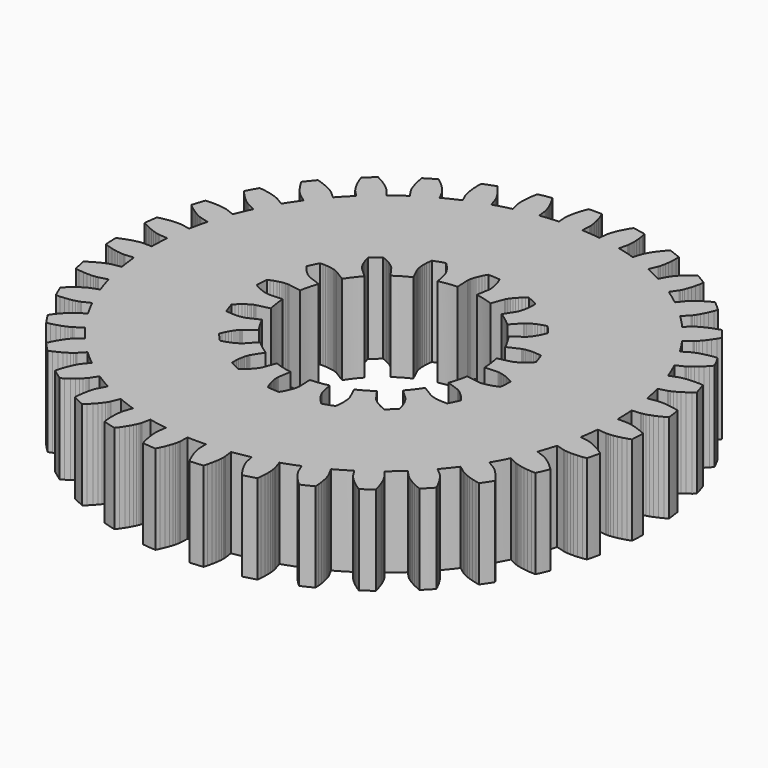
from build123d import *

# Parameters (mm, degrees)
F1_DEPTH = 5


# Not quite as in the source:
# - ends of sketch curves that miss each other by under 0.0002 mm in the source are joined


with BuildPart() as f1:
    # F0 (on Top) → F1 (new body)
    with BuildSketch(Plane.XY):
        with BuildLine():
            Line((10.175022, 8.940518), (9.814956, 8.623606))
            ThreePointArc((9.814956, 8.623606), (9.4680953178, 9.0024281141), (9.1066227348, 9.3673337267))
            Line((9.1066227348, 9.3673337267), (9.440701, 9.711531))
            Line((9.440701, 9.711531), (9.452089, 9.724074))
            Line((9.452089, 9.724074), (9.484545, 9.763184))
            Line((9.484545, 9.763184), (9.535389, 9.830931))
            Line((9.535389, 9.830931), (9.601788, 9.929185))
            Line((9.601788, 9.929185), (9.680771, 10.059599))
            Line((9.680771, 10.059599), (9.769248, 10.223605))
            Line((9.769248, 10.223605), (9.864016, 10.422403))
            Line((9.864016, 10.422403), (9.961783, 10.656955))
            Line((9.961783, 10.656955), (10.035983, 10.863432))
            ThreePointArc((10.035983, 10.863432), (9.7595522621, 11.1120973665), (9.4769619966, 11.3537399959))
            Line((9.4769619966, 11.3537399959), (9.281924, 11.253248))
            Line((9.281924, 11.253248), (9.062124, 11.125729))
            Line((9.062124, 11.125729), (8.877382, 11.005845))
            Line((8.877382, 11.005845), (8.726315, 10.896737))
            Line((8.726315, 10.896737), (8.607314, 10.801421))
            Line((8.607314, 10.801421), (8.518558, 10.722776))
            Line((8.518558, 10.722776), (8.45802, 10.663532))
            Line((8.45802, 10.663532), (8.423477, 10.626253))
            Line((8.423477, 10.626253), (8.412526, 10.613326))
            Line((8.412526, 10.613326), (8.114834, 10.237215))
            ThreePointArc((8.114834, 10.237215), (7.7059057986, 10.5480145502), (7.285085742, 10.8425126154))
            Line((7.285085742, 10.8425126154), (7.552337, 11.240831))
            Line((7.552337, 11.240831), (7.561302, 11.255206))
            Line((7.561302, 11.255206), (7.586253, 11.299482))
            Line((7.586253, 11.299482), (7.624183, 11.375219))
            Line((7.624183, 11.375219), (7.671971, 11.48375))
            Line((7.671971, 11.48375), (7.726399, 11.626171))
            Line((7.726399, 11.626171), (7.784169, 11.80334))
            Line((7.784169, 11.80334), (7.841917, 12.015864))
            Line((7.841917, 12.015864), (7.896232, 12.264104))
            Line((7.896232, 12.264104), (7.932372, 12.480512))
            ThreePointArc((7.932372, 12.480512), (7.6159827615, 12.6758223102), (7.2947870577, 12.8631231018))
            Line((7.2947870577, 12.8631231018), (7.120826, 12.72942))
            Line((7.120826, 12.72942), (6.927328, 12.564704))
            Line((6.927328, 12.564704), (6.766962, 12.41376))
            Line((6.766962, 12.41376), (6.637804, 12.279431))
            Line((6.637804, 12.279431), (6.537735, 12.164398))
            Line((6.537735, 12.164398), (6.464448, 12.07117))
            Line((6.464448, 12.07117), (6.415461, 12.002068))
            Line((6.415461, 12.002068), (6.38813, 11.95922))
            Line((6.38813, 11.95922), (6.379663, 11.944546))
            Line((6.379663, 11.944546), (6.153912, 11.521324))
            ThreePointArc((6.153912, 11.521324), (5.6960599686, 11.7541118719), (5.2294179645, 11.9687369187))
            Line((5.2294179645, 11.9687369187), (5.421252, 12.408373))
            Line((5.421252, 12.408373), (5.427506, 12.424118))
            Line((5.427506, 12.424118), (5.444151, 12.472138))
            Line((5.444151, 12.472138), (5.467948, 12.553431))
            Line((5.467948, 12.553431), (5.495588, 12.66875))
            Line((5.495588, 12.66875), (5.523711, 12.818601))
            Line((5.523711, 12.818601), (5.548918, 13.003238))
            Line((5.548918, 13.003238), (5.567791, 13.222658))
            Line((5.567791, 13.222658), (5.576908, 13.476607))
            Line((5.576908, 13.476607), (5.573826, 13.69599))
            ThreePointArc((5.573826, 13.69599), (5.2276470646, 13.8316685737), (4.8781689182, 13.9586077655))
            Line((4.8781689182, 13.9586077655), (4.730878, 13.795992))
            Line((4.730878, 13.795992), (4.569901, 13.599372))
            Line((4.569901, 13.599372), (4.439063, 13.422219))
            Line((4.439063, 13.422219), (4.335967, 13.266987))
            Line((4.335967, 13.266987), (4.258046, 13.135935))
            Line((4.258046, 13.135935), (4.202583, 13.031118))
            Line((4.202583, 13.031118), (4.166722, 12.95438))
            Line((4.166722, 12.95438), (4.147481, 12.90734))
            Line((4.147481, 12.90734), (4.14177, 12.891391))
            Line((4.14177, 12.891391), (3.995216, 12.43466))
            ThreePointArc((3.995216, 12.43466), (3.5031563536, 12.5819548058), (3.0056908928, 12.7098085461))
            Line((3.0056908928, 12.7098085461), (3.115942, 13.176633))
            Line((3.115942, 13.176633), (3.119284, 13.193242))
            Line((3.119284, 13.193242), (3.127087, 13.243462))
            Line((3.127087, 13.243462), (3.135986, 13.327697))
            Line((3.135986, 13.327697), (3.142591, 13.446099))
            Line((3.142591, 13.446099), (3.143506, 13.598563))
            Line((3.143506, 13.598563), (3.135339, 13.784734))
            Line((3.135339, 13.784734), (3.11473, 14.003998))
            Line((3.11473, 14.003998), (3.078356, 14.255493))
            Line((3.078356, 14.255493), (3.036151, 14.470801))
            ThreePointArc((3.036151, 14.470801), (2.6713088383, 14.5424859858), (2.3047810753, 14.6049834777))
            Line((2.3047810753, 14.6049834777), (2.188894, 14.418681))
            Line((2.188894, 14.418681), (2.065611, 14.196477))
            Line((2.065611, 14.196477), (1.968508, 13.998809))
            Line((1.968508, 13.998809), (1.894786, 13.827663))
            Line((1.894786, 13.827663), (1.841518, 13.684804))
            Line((1.841518, 13.684804), (1.805662, 13.571769))
            Line((1.805662, 13.571769), (1.784079, 13.48986))
            Line((1.784079, 13.48986), (1.773547, 13.440141))
            Line((1.773547, 13.440141), (1.770775, 13.423428))
            Line((1.770775, 13.423428), (1.708129, 12.947869))
            ThreePointArc((1.708129, 12.947869), (1.197676295, 13.0049359248), (0.6853760059, 13.0419091124))
            Line((0.6853760059, 13.0419091124), (0.710501, 13.520918))
            Line((0.710501, 13.520918), (0.710824, 13.537856))
            Line((0.710824, 13.537856), (0.709534, 13.588662))
            Line((0.709534, 13.588662), (0.703249, 13.673133))
            Line((0.703249, 13.673133), (0.688607, 13.790811))
            Line((0.688607, 13.790811), (0.662283, 13.940989))
            Line((0.662283, 13.940989), (0.621006, 14.122709))
            Line((0.621006, 14.122709), (0.561577, 14.33477))
            Line((0.561577, 14.33477), (0.480881, 14.575729))
            Line((0.480881, 14.575729), (0.400909, 14.78004))
            ThreePointArc((0.400909, 14.78004), (0.0291305244, 14.7854284308), (-0.3426659885, 14.7814755044))
            Line((-0.3426659885, 14.7814755044), (-0.423425, 14.577474))
            Line((-0.423425, 14.577474), (-0.505051, 14.336829))
            Line((-0.505051, 14.336829), (-0.565298, 14.124999))
            Line((-0.565298, 14.124999), (-0.607276, 13.94344))
            Line((-0.607276, 13.94344), (-0.63418, 13.793365))
            Line((-0.63418, 13.793365), (-0.649276, 13.675744))
            Line((-0.649276, 13.675744), (-0.655887, 13.591298))
            Line((-0.655887, 13.591298), (-0.657373, 13.540497))
            Line((-0.657373, 13.540497), (-0.657115, 13.523557))
            Line((-0.657115, 13.523557), (-0.63384, 13.044455))
            ThreePointArc((-0.63384, 13.044455), (-1.1462789677, 13.0094602448), (-1.6569479451, 12.9543645706))
            Line((-1.6569479451, 12.9543645706), (-1.717758, 13.430161))
            Line((-1.717758, 13.430161), (-1.720465, 13.446885))
            Line((-1.720465, 13.446885), (-1.730806, 13.496645))
            Line((-1.730806, 13.496645), (-1.752072, 13.578636))
            Line((-1.752072, 13.578636), (-1.787491, 13.691808))
            Line((-1.787491, 13.691808), (-1.840208, 13.834872))
            Line((-1.840208, 13.834872), (-1.913269, 14.006302))
            Line((-1.913269, 14.006302), (-2.009608, 14.204343))
            Line((-2.009608, 14.204343), (-2.132032, 14.427021))
            Line((-2.132032, 14.427021), (-2.247199, 14.61377))
            ThreePointArc((-2.247199, 14.61377), (-2.6139651037, 14.552687637), (-2.9790810776, 14.4824113773))
            Line((-2.9790810776, 14.4824113773), (-3.022117, 14.267268))
            Line((-3.022117, 14.267268), (-3.059462, 14.015915))
            Line((-3.059462, 14.015915), (-3.080918, 13.796732))
            Line((-3.080918, 13.796732), (-3.089802, 13.610595))
            Line((-3.089802, 13.610595), (-3.089477, 13.458128))
            Line((-3.089477, 13.458128), (-3.083328, 13.339702))
            Line((-3.083328, 13.339702), (-3.074755, 13.255432))
            Line((-3.074755, 13.255432), (-3.067145, 13.205183))
            Line((-3.067145, 13.205183), (-3.063867, 13.188561))
            Line((-3.063867, 13.188561), (-2.95542, 12.721315))
            ThreePointArc((-2.95542, 12.721315), (-3.4533751691, 12.595382232), (-3.9459998274, 12.4499884548))
            Line((-3.9459998274, 12.4499884548), (-4.090789, 12.907281))
            Line((-4.090789, 12.907281), (-4.096438, 12.923253))
            Line((-4.096438, 12.923253), (-4.115498, 12.970366))
            Line((-4.115498, 12.970366), (-4.151063, 13.047242))
            Line((-4.151063, 13.047242), (-4.20612, 13.152272))
            Line((-4.20612, 13.152272), (-4.283535, 13.283624))
            Line((-4.283535, 13.283624), (-4.386031, 13.439253))
            Line((-4.386031, 13.439253), (-4.516184, 13.61691))
            Line((-4.516184, 13.61691), (-4.676401, 13.81415))
            Line((-4.676401, 13.81415), (-4.823063, 13.977333))
            ThreePointArc((-4.823063, 13.977333), (-5.1730282225, 13.8517440222), (-5.5197280986, 13.7174032452))
            Line((-5.5197280986, 13.7174032452), (-5.523658, 13.498033))
            Line((-5.523658, 13.498033), (-5.515521, 13.244051))
            Line((-5.515521, 13.244051), (-5.497495, 13.024559))
            Line((-5.497495, 13.024559), (-5.473001, 12.839827))
            Line((-5.473001, 12.839827), (-5.445457, 12.689868))
            Line((-5.445457, 12.689868), (-5.418262, 12.574443))
            Line((-5.418262, 12.574443), (-5.394779, 12.493059))
            Line((-5.394779, 12.493059), (-5.378319, 12.444975))
            Line((-5.378319, 12.444975), (-5.372126, 12.429207))
            Line((-5.372126, 12.429207), (-5.181991, 11.988833))
            ThreePointArc((-5.181991, 11.988833), (-5.6494579891, 11.7760109862), (-6.1082050738, 11.5449921396))
            Line((-6.1082050738, 11.5449921396), (-6.33232, 11.969083))
            Line((-6.33232, 11.969083), (-6.340731, 11.983789))
            Line((-6.340731, 11.983789), (-6.367896, 12.026742))
            Line((-6.367896, 12.026742), (-6.416616, 12.096033))
            Line((-6.416616, 12.096033), (-6.489543, 12.189544))
            Line((-6.489543, 12.189544), (-6.589167, 12.304962))
            Line((-6.589167, 12.304962), (-6.717805, 12.439788))
            Line((-6.717805, 12.439788), (-6.877588, 12.59135))
            Line((-6.877588, 12.59135), (-7.070449, 12.756812))
            Line((-7.070449, 12.756812), (-7.243891, 12.891186))
            ThreePointArc((-7.243891, 12.891186), (-7.5658077628, 12.7051265282), (-7.8829488792, 12.5110388081))
            Line((-7.8829488792, 12.5110388081), (-7.847645, 12.294493))
            Line((-7.847645, 12.294493), (-7.794289, 12.046045))
            Line((-7.794289, 12.046045), (-7.737361, 11.833299))
            Line((-7.737361, 11.833299), (-7.680276, 11.655909))
            Line((-7.680276, 11.655909), (-7.626398, 11.513279))
            Line((-7.626398, 11.513279), (-7.579029, 11.404564))
            Line((-7.579029, 11.404564), (-7.541392, 11.328681))
            Line((-7.541392, 11.328681), (-7.516612, 11.284309))
            Line((-7.516612, 11.284309), (-7.507702, 11.2699))
            Line((-7.507702, 11.2699), (-7.241991, 10.870553))
            ThreePointArc((-7.241991, 10.870553), (-7.6639444746, 10.5776816964), (-8.0740691019, 10.2684631297))
            Line((-8.0740691019, 10.2684631297), (-8.370307, 10.645721))
            Line((-8.370307, 10.645721), (-8.381209, 10.658689))
            Line((-8.381209, 10.658689), (-8.415607, 10.696101))
            Line((-8.415607, 10.696101), (-8.475917, 10.755579))
            Line((-8.475917, 10.755579), (-8.564368, 10.834565))
            Line((-8.564368, 10.834565), (-8.683, 10.93034))
            Line((-8.683, 10.93034), (-8.833645, 11.040031))
            Line((-8.833645, 11.040031), (-9.017923, 11.160627))
            Line((-9.017923, 11.160627), (-9.237229, 11.288993))
            Line((-9.237229, 11.288993), (-9.431877, 11.390238))
            ThreePointArc((-9.431877, 11.390238), (-9.7153981255, 11.1496881714), (-9.9927868685, 10.9020918563))
            Line((-9.9927868685, 10.9020918563), (-9.919384, 10.69533))
            Line((-9.919384, 10.69533), (-9.822524, 10.460402))
            Line((-9.822524, 10.460402), (-9.728524, 10.26124))
            Line((-9.728524, 10.26124), (-9.640681, 10.096893))
            Line((-9.640681, 10.096893), (-9.562201, 9.966175))
            Line((-9.562201, 9.966175), (-9.496183, 9.867666))
            Line((-9.496183, 9.867666), (-9.445601, 9.799723))
            Line((-9.445601, 9.799723), (-9.413296, 9.760488))
            Line((-9.413296, 9.760488), (-9.401957, 9.747901))
            Line((-9.401957, 9.747901), (-9.069209, 9.402417))
            ThreePointArc((-9.069209, 9.402417), (-9.4320875894, 9.038909449), (-9.7804084177, 8.6614293705))
            Line((-9.7804084177, 8.6614293705), (-10.139248, 8.979729))
            Line((-10.139248, 8.979729), (-10.152289, 8.990542))
            Line((-10.152289, 8.990542), (-10.192815, 9.021211))
            Line((-10.192815, 9.021211), (-10.262776, 9.068964))
            Line((-10.262776, 9.068964), (-10.36391, 9.130888))
            Line((-10.36391, 9.130888), (-10.497736, 9.203941))
            Line((-10.497736, 9.203941), (-10.665546, 9.28497))
            Line((-10.665546, 9.28497), (-10.868396, 9.370724))
            Line((-10.868396, 9.370724), (-11.107098, 9.457869))
            Line((-11.107098, 9.457869), (-11.316696, 9.522731))
            ThreePointArc((-11.316696, 9.522731), (-11.5527092579, 9.2354223258), (-11.7814302901, 8.9422752205))
            Line((-11.7814302901, 8.9422752205), (-11.672288, 8.751942))
            Line((-11.672288, 8.751942), (-11.535036, 8.538085))
            Line((-11.535036, 8.538085), (-11.406985, 8.358908))
            Line((-11.406985, 8.358908), (-11.291209, 8.212888))
            Line((-11.291209, 8.212888), (-11.19065, 8.098283))
            Line((-11.19065, 8.098283), (-11.108103, 8.013145))
            Line((-11.108103, 8.013145), (-11.046202, 7.955325))
            Line((-11.046202, 7.955325), (-11.007411, 7.92249))
            Line((-11.007411, 7.92249), (-10.994006, 7.91213))
            Line((-10.994006, 7.91213), (-10.604918, 7.631612))
            ThreePointArc((-10.604918, 7.631612), (-10.8970576132, 7.2091516286), (-11.1723789546, 6.7755429724))
            Line((-11.1723789546, 6.7755429724), (-11.582286, 7.024654))
            Line((-11.582286, 7.024654), (-11.597049, 7.032965))
            Line((-11.597049, 7.032965), (-11.6424, 7.055905))
            Line((-11.6424, 7.055905), (-11.719763, 7.090399))
            Line((-11.719763, 7.090399), (-11.830328, 7.133269))
            Line((-11.830328, 7.133269), (-11.975048, 7.181253))
            Line((-11.975048, 7.181253), (-12.15463, 7.231016))
            Line((-12.15463, 7.231016), (-12.369531, 7.279171))
            Line((-12.369531, 7.279171), (-12.619958, 7.322294))
            Line((-12.619958, 7.322294), (-12.83777, 7.348688))
            ThreePointArc((-12.83777, 7.348688), (-13.0186887804, 7.0238547555), (-13.191390549, 6.6945792792))
            Line((-13.191390549, 6.6945792792), (-13.050018, 6.526793))
            Line((-13.050018, 6.526793), (-12.876785, 6.34088))
            Line((-12.876785, 6.34088), (-12.718799, 6.187447))
            Line((-12.718799, 6.187447), (-12.578811, 6.064445))
            Line((-12.578811, 6.064445), (-12.459404, 5.969638))
            Line((-12.459404, 5.969638), (-12.362981, 5.900608))
            Line((-12.362981, 5.900608), (-12.291751, 5.85477))
            Line((-12.291751, 5.85477), (-12.24772, 5.829389))
            Line((-12.24772, 5.829389), (-12.232681, 5.821589))
            Line((-12.232681, 5.821589), (-11.799757, 5.615053))
            ThreePointArc((-11.799757, 5.615053), (-12.0117690984, 5.1472181887), (-12.2052421698, 4.6714170652))
            Line((-12.2052421698, 4.6714170652), (-12.653043, 4.843333))
            Line((-12.653043, 4.843333), (-12.669052, 4.848875))
            Line((-12.669052, 4.848875), (-12.71777, 4.863348))
            Line((-12.71777, 4.863348), (-12.800049, 4.883474))
            Line((-12.800049, 4.883474), (-12.916492, 4.905913))
            Line((-12.916492, 4.905913), (-13.067454, 4.927285))
            Line((-13.067454, 4.927285), (-13.253036, 4.944183))
            Line((-13.253036, 4.944183), (-13.473082, 4.953192))
            Line((-13.473082, 4.953192), (-13.727184, 4.950907))
            Line((-13.727184, 4.950907), (-13.946208, 4.937985))
            ThreePointArc((-13.946208, 4.937985), (-14.0662185352, 4.5860678187), (-14.1773505157, 4.231246855))
            Line((-14.1773505157, 4.231246855), (-14.00829, 4.0914))
            Line((-14.00829, 4.0914), (-13.804646, 3.939406))
            Line((-13.804646, 3.939406), (-13.621802, 3.816648))
            Line((-13.621802, 3.816648), (-13.4621, 3.72062))
            Line((-13.4621, 3.72062), (-13.327684, 3.648657))
            Line((-13.327684, 3.648657), (-13.220485, 3.597953))
            Line((-13.220485, 3.597953), (-13.142215, 3.56557))
            Line((-13.142215, 3.56557), (-13.09436, 3.548459))
            Line((-13.09436, 3.548459), (-13.07817, 3.543469))
            Line((-13.07817, 3.543469), (-12.615324, 3.417554))
            ThreePointArc((-12.615324, 3.417554), (-12.7403942012, 2.9193816084), (-12.8458004636, 2.4166810877))
            Line((-12.8458004636, 2.4166810877), (-13.317101, 2.505877))
            Line((-13.317101, 2.505877), (-13.333843, 2.50847))
            Line((-13.333843, 2.50847), (-13.384363, 2.514012))
            Line((-13.384363, 2.514012), (-13.468913, 2.519123))
            Line((-13.468913, 2.519123), (-13.587491, 2.52041))
            Line((-13.587491, 2.52041), (-13.739844, 2.514483))
            Line((-13.739844, 2.514483), (-13.92546, 2.497973))
            Line((-13.92546, 2.497973), (-14.143579, 2.467547))
            Line((-14.143579, 2.467547), (-14.393189, 2.419926))
            Line((-14.393189, 2.419926), (-14.606386, 2.368104))
            ThreePointArc((-14.606386, 2.368104), (-14.6616304747, 2.0004133661), (-14.7076208142, 1.6314509792))
            Line((-14.7076208142, 1.6314509792), (-14.516307, 1.524038))
            Line((-14.516307, 1.524038), (-14.288796, 1.410849))
            Line((-14.288796, 1.410849), (-14.08697, 1.322712))
            Line((-14.08697, 1.322712), (-13.912689, 1.256742))
            Line((-13.912689, 1.256742), (-13.767584, 1.209937))
            Line((-13.767584, 1.209937), (-13.653053, 1.179189))
            Line((-13.653053, 1.179189), (-13.570259, 1.161302))
            Line((-13.570259, 1.161302), (-13.520118, 1.153011))
            Line((-13.520118, 1.153011), (-13.503297, 1.150993))
            Line((-13.503297, 1.150993), (-13.025407, 1.109745))
            ThreePointArc((-13.025407, 1.109745), (-13.0595144169, 0.5972460826), (-13.0734661066, 0.0838030008))
            Line((-13.0734661066, 0.0838030008), (-13.553119, 0.087411))
            Line((-13.553119, 0.087411), (-13.570055, 0.086974))
            Line((-13.570055, 0.086974), (-13.620753, 0.083407))
            Line((-13.620753, 0.083407), (-13.704856, 0.073338))
            Line((-13.704856, 0.073338), (-13.821759, 0.053431))
            Line((-13.821759, 0.053431), (-13.970605, 0.020396))
            Line((-13.970605, 0.020396), (-14.15029, -0.028992))
            Line((-14.15029, -0.028992), (-14.359471, -0.097876))
            Line((-14.359471, -0.097876), (-14.596567, -0.189301))
            Line((-14.596567, -0.189301), (-14.797085, -0.278358))
            ThreePointArc((-14.797085, -0.278358), (-14.7857874955, -0.6500040317), (-14.7651579616, -1.0212489974))
            Line((-14.7651579616, -1.0212489974), (-14.557739, -1.092775))
            Line((-14.557739, -1.092775), (-14.313673, -1.163521))
            Line((-14.313673, -1.163521), (-14.099354, -1.214205))
            Line((-14.099354, -1.214205), (-13.916094, -1.247995))
            Line((-13.916094, -1.247995), (-13.764963, -1.268138))
            Line((-13.764963, -1.268138), (-13.646783, -1.277942))
            Line((-13.646783, -1.277942), (-13.562126, -1.280758))
            Line((-13.562126, -1.280758), (-13.51131, -1.279963))
            Line((-13.51131, -1.279963), (-13.494399, -1.278946))
            Line((-13.494399, -1.278946), (-13.016823, -1.234199))
            ThreePointArc((-13.016823, -1.234199), (-12.9588730132, -1.7445519941), (-12.880921728, -2.2522349527))
            Line((-12.880921728, -2.2522349527), (-13.353511, -2.334331))
            Line((-13.353511, -2.334331), (-13.370097, -2.337785))
            Line((-13.370097, -2.337785), (-13.419342, -2.350347))
            Line((-13.419342, -2.350347), (-13.500297, -2.375271))
            Line((-13.500297, -2.375271), (-13.611766, -2.415732))
            Line((-13.611766, -2.415732), (-13.752321, -2.474814))
            Line((-13.752321, -2.474814), (-13.9203, -2.555492))
            Line((-13.9203, -2.555492), (-14.11382, -2.66062))
            Line((-14.11382, -2.66062), (-14.330781, -2.792911))
            Line((-14.330781, -2.792911), (-14.512174, -2.916341))
            ThreePointArc((-14.512174, -2.916341), (-14.4346989596, -3.2799969988), (-14.3481127103, -3.6415919268))
            Line((-14.3481127103, -3.6415919268), (-14.131256, -3.674933))
            Line((-14.131256, -3.674933), (-13.87848, -3.700963))
            Line((-13.87848, -3.700963), (-13.658555, -3.712563))
            Line((-13.658555, -3.712563), (-13.472207, -3.713088))
            Line((-13.472207, -3.713088), (-13.319908, -3.705922))
            Line((-13.319908, -3.705922), (-13.201876, -3.694467))
            Line((-13.201876, -3.694467), (-13.118077, -3.682121))
            Line((-13.118077, -3.682121), (-13.068219, -3.672265))
            Line((-13.068219, -3.672265), (-13.051762, -3.668245))
            Line((-13.051762, -3.668245), (-12.589851, -3.538943))
            ThreePointArc((-12.589851, -3.538943), (-12.4417046023, -4.0307471058), (-12.2743556439, -4.5163528694))
            Line((-12.2743556439, -4.5163528694), (-12.724692, -4.681513))
            Line((-12.724692, -4.681513), (-12.740394, -4.687873))
            Line((-12.740394, -4.687873), (-12.786605, -4.709027))
            Line((-12.786605, -4.709027), (-12.861808, -4.748005))
            Line((-12.861808, -4.748005), (-12.964262, -4.807719))
            Line((-12.964262, -4.807719), (-13.092008, -4.890949))
            Line((-13.092008, -4.890949), (-13.242882, -5.000325))
            Line((-13.242882, -5.000325), (-13.414521, -5.138317))
            Line((-13.414521, -5.138317), (-13.604374, -5.307222))
            Line((-13.604374, -5.307222), (-13.760813, -5.461057))
            ThreePointArc((-13.760813, -5.461057), (-13.6196492767, -5.8050353693), (-13.4698891049, -6.1453590477))
            Line((-13.4698891049, -6.1453590477), (-13.250564, -6.139443))
            Line((-13.250564, -6.139443), (-12.997203, -6.119919))
            Line((-12.997203, -6.119919), (-12.77874, -6.092064))
            Line((-12.77874, -6.092064), (-12.595293, -6.059307))
            Line((-12.595293, -6.059307), (-12.446721, -6.025063))
            Line((-12.446721, -6.025063), (-12.332632, -5.992716))
            Line((-12.332632, -5.992716), (-12.252384, -5.965605))
            Line((-12.252384, -5.965605), (-12.205087, -5.947006))
            Line((-12.205087, -5.947006), (-12.189612, -5.940111))
            Line((-12.189612, -5.940111), (-11.758212, -5.73041))
            ThreePointArc((-11.758212, -5.73041), (-11.5246315753, -6.187857722), (-11.2732639309, -6.6357779594))
            Line((-11.2732639309, -6.6357779594), (-11.686872, -6.878695))
            Line((-11.686872, -6.878695), (-11.701186, -6.887757))
            Line((-11.701186, -6.887757), (-11.742878, -6.916822))
            Line((-11.742878, -6.916822), (-11.809912, -6.968602))
            Line((-11.809912, -6.968602), (-11.900057, -7.04565))
            Line((-11.900057, -7.04565), (-12.01089, -7.150352))
            Line((-12.01089, -7.150352), (-12.139809, -7.28491))
            Line((-12.139809, -7.28491), (-12.28405, -7.451332))
            Line((-12.28405, -7.451332), (-12.440693, -7.651422))
            Line((-12.440693, -7.651422), (-12.567149, -7.830718))
            ThreePointArc((-12.567149, -7.830718), (-12.3668345135, -8.1439630449), (-12.1587138721, -8.4520769113))
            Line((-12.1587138721, -8.4520769113), (-11.94397, -8.407093))
            Line((-11.94397, -8.407093), (-11.698166, -8.342644))
            Line((-11.698166, -8.342644), (-11.488189, -8.276229))
            Line((-11.488189, -8.276229), (-11.313538, -8.211242))
            Line((-11.313538, -8.211242), (-11.173469, -8.15102))
            Line((-11.173469, -8.15102), (-11.066989, -8.098822))
            Line((-11.066989, -8.098822), (-10.992871, -8.057818))
            Line((-10.992871, -8.057818), (-10.949655, -8.031072))
            Line((-10.949655, -8.031072), (-10.93566, -8.021525))
            Line((-10.93566, -8.021525), (-10.548636, -7.738164))
            ThreePointArc((-10.548636, -7.738164), (-10.2371291534, -8.1465532386), (-9.9098218023, -8.5423918299))
            Line((-9.9098218023, -8.5423918299), (-10.273409, -8.855257))
            Line((-10.273409, -8.855257), (-10.285875, -8.866729))
            Line((-10.285875, -8.866729), (-10.321706, -8.902772))
            Line((-10.321706, -8.902772), (-10.378418, -8.965689))
            Line((-10.378418, -8.965689), (-10.453357, -9.057595))
            Line((-10.453357, -9.057595), (-10.543713, -9.180405))
            Line((-10.543713, -9.180405), (-10.646534, -9.335819))
            Line((-10.646534, -9.335819), (-10.758741, -9.525322))
            Line((-10.758741, -9.525322), (-10.877139, -9.750166))
            Line((-10.877139, -9.750166), (-10.969549, -9.949161))
            ThreePointArc((-10.969549, -9.949161), (-10.7165215888, -10.2216041293), (-10.4567298923, -10.4876048921))
            Line((-10.4567298923, -10.4876048921), (-10.253469, -10.405))
            Line((-10.253469, -10.405), (-10.023123, -10.297697))
            Line((-10.023123, -10.297697), (-9.828379, -10.194856))
            Line((-9.828379, -10.194856), (-9.668139, -10.099729))
            Line((-9.668139, -10.099729), (-9.541073, -10.015464))
            Line((-9.541073, -10.015464), (-9.445625, -9.945092))
            Line((-9.445625, -9.945092), (-9.38002, -9.891513))
            Line((-9.38002, -9.891513), (-9.342274, -9.85748))
            Line((-9.342274, -9.85748), (-9.330209, -9.845587))
            Line((-9.330209, -9.845587), (-9, -9.497675))
            ThreePointArc((-9, -9.497675), (-8.620578636, -9.8438794307), (-8.227851686, -10.1749136123))
            Line((-8.227851686, -10.1749136123), (-8.529731, -10.547672))
            Line((-8.529731, -10.547672), (-8.539949, -10.561186))
            Line((-8.539949, -10.561186), (-8.568769, -10.603047))
            Line((-8.568769, -10.603047), (-8.613335, -10.675079))
            Line((-8.613335, -10.675079), (-8.670659, -10.778889))
            Line((-8.670659, -10.778889), (-8.737635, -10.915859))
            Line((-8.737635, -10.915859), (-8.811053, -11.087135))
            Line((-8.811053, -11.087135), (-8.88762, -11.293628))
            Line((-8.88762, -11.293628), (-8.963968, -11.535999))
            Line((-8.963968, -11.535999), (-9.019361, -11.748297))
            ThreePointArc((-9.019361, -11.748297), (-8.7217524774, -11.9711821257), (-8.4186389377, -12.1865209099))
            Line((-8.4186389377, -12.1865209099), (-8.233395, -12.06895))
            Line((-8.233395, -12.06895), (-8.02591, -11.922241))
            Line((-8.02591, -11.922241), (-7.852659, -11.78628))
            Line((-7.852659, -11.78628), (-7.71198, -11.66407))
            Line((-7.71198, -11.66407), (-7.602002, -11.55847))
            Line((-7.602002, -11.55847), (-7.520653, -11.472186))
            Line((-7.520653, -11.472186), (-7.465669, -11.407754))
            Line((-7.465669, -11.407754), (-7.434607, -11.367528))
            Line((-7.434607, -11.367528), (-7.424859, -11.353672))
            Line((-7.424859, -11.353672), (-7.162079, -10.95239))
            ThreePointArc((-7.162079, -10.95239), (-6.7269374664, -11.2252825742), (-6.2814129926, -11.4808729864))
            Line((-6.2814129926, -11.4808729864), (-6.511883, -11.901544))
            Line((-6.511883, -11.901544), (-6.519524, -11.916664))
            Line((-6.519524, -11.916664), (-6.540406, -11.962999))
            Line((-6.540406, -11.962999), (-6.571394, -12.041831))
            Line((-6.571394, -12.041831), (-6.609261, -12.154209))
            Line((-6.609261, -12.154209), (-6.650703, -12.300936))
            Line((-6.650703, -12.300936), (-6.692359, -12.482569))
            Line((-6.692359, -12.482569), (-6.730825, -12.699415))
            Line((-6.730825, -12.699415), (-6.762669, -12.951524))
            Line((-6.762669, -12.951524), (-6.779264, -13.1703))
            ThreePointArc((-6.779264, -13.1703), (-6.4466411712, -13.336463737), (-6.1099488992, -13.4942187776))
            Line((-6.1099488992, -13.4942187776), (-5.948674, -13.34546))
            Line((-5.948674, -13.34546), (-5.77072, -13.164062))
            Line((-5.77072, -13.164062), (-5.624529, -12.999351))
            Line((-5.624529, -12.999351), (-5.507933, -12.853985))
            Line((-5.507933, -12.853985), (-5.418578, -12.730445))
            Line((-5.418578, -12.730445), (-5.353943, -12.631022))
            Line((-5.353943, -12.631022), (-5.311347, -12.557807))
            Line((-5.311347, -12.557807), (-5.287967, -12.512682))
            Line((-5.287967, -12.512682), (-5.28085, -12.497308))
            Line((-5.28085, -12.497308), (-5.093945, -12.055554))
            ThreePointArc((-5.093945, -12.055554), (-4.6170691765, -12.2463631291), (-4.1330668942, -12.4182946824))
            Line((-4.1330668942, -12.4182946824), (-4.28472, -12.873357))
            Line((-4.28472, -12.873357), (-4.289538, -12.889599))
            Line((-4.289538, -12.889599), (-4.301811, -12.938917))
            Line((-4.301811, -12.938917), (-4.318225, -13.022016))
            Line((-4.318225, -13.022016), (-4.335417, -13.139349))
            Line((-4.335417, -13.139349), (-4.349995, -13.291118))
            Line((-4.349995, -13.291118), (-4.358549, -13.477271))
            Line((-4.358549, -13.477271), (-4.357677, -13.6975))
            Line((-4.357677, -13.6975), (-4.343994, -13.951243))
            Line((-4.343994, -13.951243), (-4.321259, -14.169467))
            ThreePointArc((-4.321259, -14.169467), (-3.9643117262, -14.2735678262), (-3.6048619905, -14.3686689621))
            Line((-3.6048619905, -14.3686689621), (-3.472741, -14.193505))
            Line((-3.472741, -14.193505), (-3.330036, -13.983246))
            Line((-3.330036, -13.983246), (-3.215605, -13.795079))
            Line((-3.215605, -13.795079), (-3.126838, -13.63123))
            Line((-3.126838, -13.63123), (-3.060979, -13.49372))
            Line((-3.060979, -13.49372), (-3.015135, -13.384354))
            Line((-3.015135, -13.384354), (-2.986297, -13.30471))
            Line((-2.986297, -13.30471), (-2.97135, -13.256135))
            Line((-2.97135, -13.256135), (-2.967091, -13.239738))
            Line((-2.967091, -13.239738), (-2.862069, -12.771709))
            ThreePointArc((-2.862069, -12.771709), (-2.358786646, -12.8743029359), (-1.851862935, -12.9570495461))
            Line((-1.851862935, -12.9570495461), (-1.919824, -13.431878))
            Line((-1.919824, -13.431878), (-1.921664, -13.448719))
            Line((-1.921664, -13.448719), (-1.924934, -13.499436))
            Line((-1.924934, -13.499436), (-1.926246, -13.58413))
            Line((-1.926246, -13.58413), (-1.922212, -13.702647))
            Line((-1.922212, -13.702647), (-1.909456, -13.85458))
            Line((-1.909456, -13.85458), (-1.884634, -14.039269))
            Line((-1.884634, -14.039269), (-1.844453, -14.255803))
            Line((-1.844453, -14.255803), (-1.785681, -14.503025))
            Line((-1.785681, -14.503025), (-1.724346, -14.713683))
            ThreePointArc((-1.724346, -14.713683), (-1.3545471379, -14.7523753806), (-0.9838929973, -14.7817659602))
            Line((-0.9838929973, -14.7817659602), (-0.885172, -14.585825))
            Line((-0.885172, -14.585825), (-0.782304, -14.353465))
            Line((-0.782304, -14.353465), (-0.703311, -14.147889))
            Line((-0.703311, -14.147889), (-0.645227, -13.970823))
            Line((-0.645227, -13.970823), (-0.604979, -13.823764))
            Line((-0.604979, -13.823764), (-0.5794, -13.70797))
            Line((-0.5794, -13.70797), (-0.565246, -13.624456))
            Line((-0.565246, -13.624456), (-0.559212, -13.573993))
            Line((-0.559212, -13.573993), (-0.557951, -13.557099))
            Line((-0.557951, -13.557099), (-0.538185, -13.077839))
            ThreePointArc((-0.538185, -13.077839), (-0.0246719852, -13.0889196449), (0.4888799909, -13.0798217564))
            Line((0.4888799909, -13.0798217564), (0.506795, -13.559154))
            Line((0.506795, -13.559154), (0.507991, -13.576053))
            Line((0.507991, -13.576053), (0.51383, -13.626539))
            Line((0.51383, -13.626539), (0.527661, -13.710107))
            Line((0.527661, -13.710107), (0.552793, -13.825999))
            Line((0.552793, -13.825999), (0.592473, -13.973212))
            Line((0.592473, -13.973212), (0.649873, -14.150501))
            Line((0.649873, -14.150501), (0.728072, -14.35638))
            Line((0.728072, -14.35638), (0.830043, -14.589136))
            Line((0.830043, -14.589136), (0.928007, -14.785456))
            ThreePointArc((0.928007, -14.785456), (1.2987717052, -14.7574967827), (1.6687170229, -14.7202322019))
            Line((1.6687170229, -14.7202322019), (1.730865, -14.509813))
            Line((1.730865, -14.509813), (1.79059, -14.262819))
            Line((1.79059, -14.262819), (1.831607, -14.046442))
            Line((1.831607, -14.046442), (1.857141, -13.861851))
            Line((1.857141, -13.861851), (1.870484, -13.709968))
            Line((1.870484, -13.709968), (1.874976, -13.591467))
            Line((1.874976, -13.591467), (1.873991, -13.506769))
            Line((1.873991, -13.506769), (1.870917, -13.456039))
            Line((1.870917, -13.456039), (1.869142, -13.439191))
            Line((1.869142, -13.439191), (1.803014, -12.964104))
            ThreePointArc((1.803014, -12.964104), (2.3102533512, -12.8833151325), (2.813928037, -12.7826651678))
            Line((2.813928037, -12.7826651678), (2.917143, -13.251096))
            Line((2.917143, -13.251096), (2.921338, -13.267509))
            Line((2.921338, -13.267509), (2.936097, -13.316142))
            Line((2.936097, -13.316142), (2.964628, -13.395896))
            Line((2.964628, -13.395896), (3.010049, -13.505439))
            Line((3.010049, -13.505439), (3.075377, -13.643201))
            Line((3.075377, -13.643201), (3.163511, -13.807392))
            Line((3.163511, -13.807392), (3.277215, -13.996))
            Line((3.277215, -13.996), (3.419106, -14.206807))
            Line((3.419106, -14.206807), (3.55055, -14.38248))
            ThreePointArc((3.55055, -14.38248), (3.9103643447, -14.2887676659), (4.2677108787, -14.1860455971))
            Line((4.2677108787, -14.1860455971), (4.291289, -13.967911))
            Line((4.291289, -13.967911), (4.305951, -13.714222))
            Line((4.305951, -13.714222), (4.307674, -13.493998))
            Line((4.307674, -13.493998), (4.299838, -13.307814))
            Line((4.299838, -13.307814), (4.285846, -13.15599))
            Line((4.285846, -13.15599), (4.269107, -13.038591))
            Line((4.269107, -13.038591), (4.253014, -12.95543))
            Line((4.253014, -12.95543), (4.240931, -12.906065))
            Line((4.240931, -12.906065), (4.236176, -12.889804))
            Line((4.236176, -12.889804), (4.086281, -12.434159))
            ThreePointArc((4.086281, -12.434159), (4.5709433693, -12.2640977789), (5.0485519074, -12.0751307787))
            Line((5.0485519074, -12.0751307787), (5.23375, -12.517603))
            Line((5.23375, -12.517603), (5.240808, -12.533005))
            Line((5.240808, -12.533005), (5.264014, -12.57822))
            Line((5.264014, -12.57822), (5.306327, -12.651599))
            Line((5.306327, -12.651599), (5.370578, -12.75127))
            Line((5.370578, -12.75127), (5.459455, -12.875154))
            Line((5.459455, -12.875154), (5.575489, -13.020969))
            Line((5.575489, -13.020969), (5.721043, -13.186243))
            Line((5.721043, -13.186243), (5.898295, -13.368327))
            Line((5.898295, -13.368327), (6.058995, -13.517707))
            ThreePointArc((6.058995, -13.517707), (6.3962938566, -13.3612529427), (6.7295559716, -13.1963749444))
            Line((6.7295559716, -13.1963749444), (6.713805, -12.977536))
            Line((6.713805, -12.977536), (6.682934, -12.725306))
            Line((6.682934, -12.725306), (6.645306, -12.508314))
            Line((6.645306, -12.508314), (6.604351, -12.326521))
            Line((6.604351, -12.326521), (6.563476, -12.179635))
            Line((6.563476, -12.179635), (6.526043, -12.067112))
            Line((6.526043, -12.067112), (6.49536, -11.98816))
            Line((6.49536, -11.98816), (6.474656, -11.941746))
            Line((6.474656, -11.941746), (6.467075, -11.926596))
            Line((6.467075, -11.926596), (6.23823, -11.505038))
            ThreePointArc((6.23823, -11.505038), (6.6847380048, -11.251169527), (7.120929943, -10.9799589122))
            Line((7.120929943, -10.9799589122), (7.382158, -11.382253))
            Line((7.382158, -11.382253), (7.391853, -11.396146))
            Line((7.391853, -11.396146), (7.422759, -11.436491))
            Line((7.422759, -11.436491), (7.477494, -11.501135))
            Line((7.477494, -11.501135), (7.55851, -11.587733))
            Line((7.55851, -11.587733), (7.668079, -11.693756))
            Line((7.668079, -11.693756), (7.808285, -11.816509))
            Line((7.808285, -11.816509), (7.98101, -11.953138))
            Line((7.98101, -11.953138), (8.187927, -12.100646))
            Line((8.187927, -12.100646), (8.372716, -12.218931))
            ThreePointArc((8.372716, -12.218931), (8.6766584879, -12.0047643665), (8.9751248387, -11.7830297884))
            Line((8.9751248387, -11.7830297884), (8.920552, -11.57052))
            Line((8.920552, -11.57052), (8.84514, -11.327856))
            Line((8.84514, -11.327856), (8.769371, -11.121069))
            Line((8.769371, -11.121069), (8.696614, -10.94951))
            Line((8.696614, -10.94951), (8.630168, -10.812284))
            Line((8.630168, -10.812284), (8.573245, -10.708253))
            Line((8.573245, -10.708253), (8.528957, -10.636049))
            Line((8.528957, -10.636049), (8.500299, -10.594077))
            Line((8.500299, -10.594077), (8.490134, -10.580524))
            Line((8.490134, -10.580524), (8.189695, -10.206603))
            ThreePointArc((8.189695, -10.206603), (8.5836973531, -9.8770871407), (8.9644529555, -9.5323499527))
            Line((8.9644529555, -9.5323499527), (9.293316, -9.881534))
            Line((9.293316, -9.881534), (9.305335, -9.893473))
            Line((9.305335, -9.893473), (9.342949, -9.927652))
            Line((9.342949, -9.927652), (9.408347, -9.981484))
            Line((9.408347, -9.981484), (9.503523, -10.052224))
            Line((9.503523, -10.052224), (9.630262, -10.136979))
            Line((9.630262, -10.136979), (9.790134, -10.232724))
            Line((9.790134, -10.232724), (9.984479, -10.336316))
            Line((9.984479, -10.336316), (10.214409, -10.444507))
            Line((10.214409, -10.444507), (10.41735, -10.527896))
            ThreePointArc((10.41735, -10.527896), (10.678166579, -10.2629001202), (10.93224396, -9.9914359635))
            Line((10.93224396, -9.9914359635), (10.840603, -9.792086))
            Line((10.840603, -9.792086), (10.723074, -9.566786))
            Line((10.723074, -9.566786), (10.611599, -9.376852))
            Line((10.611599, -9.376852), (10.509379, -9.221041))
            Line((10.509379, -9.221041), (10.419497, -9.097884))
            Line((10.419497, -9.097884), (10.344914, -9.005689))
            Line((10.344914, -9.005689), (10.288445, -8.942554))
            Line((10.288445, -8.942554), (10.252753, -8.906373))
            Line((10.252753, -8.906373), (10.240332, -8.894853))
            Line((10.240332, -8.894853), (9.877955, -8.580586))
            ThreePointArc((9.877955, -8.580586), (10.2067879994, -8.1860143104), (10.5198691556, -7.7788311149))
            Line((10.5198691556, -7.7788311149), (10.905796, -8.063683))
            Line((10.905796, -8.063683), (10.919755, -8.073284))
            Line((10.919755, -8.073284), (10.962867, -8.100197))
            Line((10.962867, -8.100197), (11.036826, -8.141486))
            Line((11.036826, -8.141486), (11.143103, -8.194095))
            Line((11.143103, -8.194095), (11.28294, -8.254858))
            Line((11.28294, -8.254858), (11.457338, -8.320519))
            Line((11.457338, -8.320519), (11.667057, -8.387744))
            Line((11.667057, -8.387744), (11.91261, -8.453141))
            Line((11.91261, -8.453141), (12.127179, -8.498953))
            ThreePointArc((12.127179, -8.498953), (12.3364877767, -8.191645233), (12.5380103234, -7.8791762029))
            Line((12.5380103234, -7.8791762029), (12.412247, -7.699393))
            Line((12.412247, -7.699393), (12.256377, -7.498699))
            Line((12.256377, -7.498699), (12.11278, -7.331722))
            Line((12.11278, -7.331722), (11.984381, -7.196668))
            Line((11.984381, -7.196668), (11.873954, -7.091539))
            Line((11.873954, -7.091539), (11.784107, -7.014143))
            Line((11.784107, -7.014143), (11.717273, -6.962105))
            Line((11.717273, -6.962105), (11.675694, -6.932879))
            Line((11.675694, -6.932879), (11.661415, -6.923762))
            Line((11.661415, -6.923762), (11.248747, -6.67925))
            ThreePointArc((11.248747, -6.67925), (11.5018422334, -6.2323035931), (11.7371868144, -5.7757609089))
            Line((11.7371868144, -5.7757609089), (12.167774, -5.987126))
            Line((12.167774, -5.987126), (12.183222, -5.99408))
            Line((12.183222, -5.99408), (12.230447, -6.012862))
            Line((12.230447, -6.012862), (12.31059, -6.040282))
            Line((12.31059, -6.040282), (12.424553, -6.073069))
            Line((12.424553, -6.073069), (12.572992, -6.107887))
            Line((12.572992, -6.107887), (12.756312, -6.141352))
            Line((12.756312, -6.141352), (12.974665, -6.17005))
            Line((12.974665, -6.17005), (13.227949, -6.190551))
            Line((13.227949, -6.190551), (13.447249, -6.197315))
            ThreePointArc((13.447249, -6.197315), (13.5983220825, -5.8575719076), (13.7408126944, -5.5141408777))
            Line((13.7408126944, -5.5141408777), (13.584969, -5.359702))
            Line((13.584969, -5.359702), (13.395769, -5.190066))
            Line((13.395769, -5.190066), (13.224665, -5.051412))
            Line((13.224665, -5.051412), (13.074214, -4.941455))
            Line((13.074214, -4.941455), (12.94679, -4.857733))
            Line((12.94679, -4.857733), (12.844567, -4.797623))
            Line((12.844567, -4.797623), (12.769515, -4.758355))
            Line((12.769515, -4.758355), (12.723386, -4.737023))
            Line((12.723386, -4.737023), (12.707709, -4.730602))
            Line((12.707709, -4.730602), (12.258013, -4.563705))
            ThreePointArc((12.258013, -4.563705), (12.4272357217, -4.078749369), (12.5772793872, -3.58752111))
            Line((12.5772793872, -3.58752111), (13.038688, -3.718605))
            Line((13.038688, -3.718605), (13.055129, -3.722689))
            Line((13.055129, -3.722689), (13.104949, -3.732737))
            Line((13.104949, -3.732737), (13.1887, -3.745406))
            Line((13.1887, -3.745406), (13.306686, -3.757317))
            Line((13.306686, -3.757317), (13.458956, -3.765071))
            Line((13.458956, -3.765071), (13.645305, -3.765265))
            Line((13.645305, -3.765265), (13.865273, -3.754513))
            Line((13.865273, -3.754513), (14.118148, -3.72946))
            Line((14.118148, -3.72946), (14.335132, -3.696957))
            ThreePointArc((14.335132, -3.696957), (14.4231134371, -3.3356985783), (14.5019921695, -2.9723440346))
            Line((14.5019921695, -2.9723440346), (14.321077, -2.848214))
            Line((14.321077, -2.848214), (14.104628, -2.715087))
            Line((14.104628, -2.715087), (13.911515, -2.609213))
            Line((13.911515, -2.609213), (13.743849, -2.527887))
            Line((13.743849, -2.527887), (13.603523, -2.468263))
            Line((13.603523, -2.468263), (13.492211, -2.427372))
            Line((13.492211, -2.427372), (13.411353, -2.402136))
            Line((13.411353, -2.402136), (13.362156, -2.389383))
            Line((13.362156, -2.389383), (13.345584, -2.385865))
            Line((13.345584, -2.385865), (12.873315, -2.301946))
            ThreePointArc((12.873315, -2.301946), (12.9532259364, -1.7945676298), (13.0131461569, -1.2844420153))
            Line((13.0131461569, -1.2844420153), (13.490545, -1.331032))
            Line((13.490545, -1.331032), (13.507452, -1.332115))
            Line((13.507452, -1.332115), (13.558265, -1.333106))
            Line((13.558265, -1.333106), (13.642933, -1.330617))
            Line((13.642933, -1.330617), (13.761149, -1.321269))
            Line((13.761149, -1.321269), (13.912357, -1.301709))
            Line((13.912357, -1.301709), (14.095746, -1.268627))
            Line((14.095746, -1.268627), (14.310259, -1.218771))
            Line((14.310259, -1.218771), (14.554596, -1.148968))
            Line((14.554596, -1.148968), (14.76229, -1.078243))
            ThreePointArc((14.76229, -1.078243), (14.7843521866, -0.7070805352), (14.7970838423, -0.3354809966))
            Line((14.7970838423, -0.3354809966), (14.596911, -0.24565))
            Line((14.596911, -0.24565), (14.36017, -0.153311))
            Line((14.36017, -0.153311), (14.151257, -0.08362))
            Line((14.151257, -0.08362), (13.971764, -0.033538))
            Line((13.971764, -0.033538), (13.823047, 7.1e-05))
            Line((13.823047, 7.1e-05), (13.706221, 0.02043))
            Line((13.706221, 0.02043), (13.622157, 0.030822))
            Line((13.622157, 0.030822), (13.571474, 0.034586))
            Line((13.571474, 0.034586), (13.55454, 0.035088))
            Line((13.55454, 0.035088), (13.074876, 0.033332))
            ThreePointArc((13.074876, 0.033332), (13.0629068222, 0.5468251785), (13.0307776595, 1.0594519719))
            Line((13.0307776595, 1.0594519719), (13.508824, 1.098854))
            Line((13.508824, 1.098854), (13.525652, 1.100807))
            Line((13.525652, 1.100807), (13.575825, 1.108905))
            Line((13.575825, 1.108905), (13.658688, 1.126472))
            Line((13.658688, 1.126472), (13.773336, 1.156778))
            Line((13.773336, 1.156778), (13.918621, 1.203022))
            Line((13.918621, 1.203022), (14.093156, 1.268319))
            Line((14.093156, 1.268319), (14.29532, 1.355676))
            Line((14.29532, 1.355676), (14.523266, 1.467986))
            Line((14.523266, 1.467986), (14.714993, 1.574659))
            ThreePointArc((14.714993, 1.574659), (14.6704278116, 1.9437960498), (14.6166032256, 2.3116970359))
            Line((14.6166032256, 2.3116970359), (14.403608, 2.364342))
            Line((14.403608, 2.364342), (14.154183, 2.412926))
            Line((14.154183, 2.412926), (13.936183, 2.444194))
            Line((13.936183, 2.444194), (13.750632, 2.461421))
            Line((13.750632, 2.461421), (13.598304, 2.467936))
            Line((13.598304, 2.467936), (13.479721, 2.467107))
            Line((13.479721, 2.467107), (13.395152, 2.462323))
            Line((13.395152, 2.462323), (13.344611, 2.456976))
            Line((13.344611, 2.456976), (13.32786, 2.454447))
            Line((13.32786, 2.454447), (12.856218, 2.367071))
            ThreePointArc((12.856218, 2.367071), (12.752753262, 2.8701751172), (12.6296073303, 3.3688270885))
            Line((12.6296073303, 3.3688270885), (13.092935, 3.492954))
            Line((13.092935, 3.492954), (13.109145, 3.497881))
            Line((13.109145, 3.497881), (13.157066, 3.514807))
            Line((13.157066, 3.514807), (13.23546, 3.546887))
            Line((13.23546, 3.546887), (13.342854, 3.597177))
            Line((13.342854, 3.597177), (13.477547, 3.668621))
            Line((13.477547, 3.668621), (13.637618, 3.764032))
            Line((13.637618, 3.764032), (13.820935, 3.886083))
            Line((13.820935, 3.886083), (14.025164, 4.03729))
            Line((14.025164, 4.03729), (14.194763, 4.176483))
            ThreePointArc((14.194763, 4.176483), (14.0850018823, 4.5317302481), (13.9663510655, 4.884108023))
            Line((13.9663510655, 4.884108023), (13.747378, 4.897876))
            Line((13.747378, 4.897876), (13.493287, 4.901142))
            Line((13.493287, 4.901142), (13.273207, 4.892982))
            Line((13.273207, 4.892982), (13.087562, 4.876801))
            Line((13.087562, 4.876801), (12.936519, 4.856012))
            Line((12.936519, 4.856012), (12.81999, 4.834022))
            Line((12.81999, 4.834022), (12.737634, 4.814214))
            Line((12.737634, 4.814214), (12.68886, 4.799929))
            Line((12.68886, 4.799929), (12.67283, 4.794449))
            Line((12.67283, 4.794449), (12.224369, 4.624263))
            ThreePointArc((12.224369, 4.624263), (12.0327340058, 5.1008074358), (11.8225294056, 5.5694571916))
            Line((11.8225294056, 5.5694571916), (12.256248, 5.77432))
            Line((12.256248, 5.77432), (12.271317, 5.782062))
            Line((12.271317, 5.782062), (12.315445, 5.807273))
            Line((12.315445, 5.807273), (12.386852, 5.852836))
            Line((12.386852, 5.852836), (12.48354, 5.921494))
            Line((12.48354, 5.921494), (12.603312, 6.015839))
            Line((12.603312, 6.015839), (12.743774, 6.138299))
            Line((12.743774, 6.138299), (12.902352, 6.291121))
            Line((12.902352, 6.291121), (13.0763, 6.476364))
            Line((13.0763, 6.476364), (13.21832, 6.643603))
            ThreePointArc((13.21832, 6.643603), (13.0468905606, 6.9735432401), (12.8672266952, 7.2990728267))
            Line((12.8672266952, 7.2990728267), (12.649315, 7.273519))
            Line((12.649315, 7.273519), (12.398724, 7.231364))
            Line((12.398724, 7.231364), (12.183638, 7.184038))
            Line((12.183638, 7.184038), (12.003866, 7.134969))
            Line((12.003866, 7.134969), (11.858961, 7.087544))
            Line((11.858961, 7.087544), (11.748231, 7.045101))
            Line((11.748231, 7.045101), (11.670736, 7.010906))
            Line((11.670736, 7.010906), (11.625297, 6.988141))
            Line((11.625297, 6.988141), (11.610502, 6.979887))
            Line((11.610502, 6.979887), (11.199636, 6.73236))
            ThreePointArc((11.199636, 6.73236), (10.9259909338, 7.1670283678), (10.6354839676, 7.5906129768))
            Line((10.6354839676, 7.5906129768), (11.025652, 7.869628))
            Line((11.025652, 7.869628), (11.039097, 7.879936))
            Line((11.039097, 7.879936), (11.078014, 7.912621))
            Line((11.078014, 7.912621), (11.140138, 7.970202))
            Line((11.140138, 7.970202), (11.223013, 8.05502))
            Line((11.223013, 8.05502), (11.324014, 8.169236))
            Line((11.324014, 8.169236), (11.440353, 8.314808))
            Line((11.440353, 8.314808), (11.569095, 8.49349))
            Line((11.569095, 8.49349), (11.707171, 8.706815))
            Line((11.707171, 8.706815), (11.817047, 8.896726))
            ThreePointArc((11.817047, 8.896726), (11.5894595579, 9.1907533743), (11.3545578236, 9.4789708525))
            Line((11.3545578236, 9.4789708525), (11.14471, 9.414919))
            Line((11.14471, 9.414919), (10.905673, 9.328696))
            Line((10.905673, 9.328696), (10.702495, 9.243726))
            Line((10.702495, 9.243726), (10.534373, 9.163345))
            Line((10.534373, 9.163345), (10.400265, 9.090809))
            Line((10.400265, 9.090809), (10.298893, 9.029276))
            Line((10.298893, 9.029276), (10.228749, 8.981794))
            Line((10.228749, 8.981794), (10.188105, 8.951281))
            Line((10.188105, 8.951281), (10.175022, 8.940518))
        make_face()
        with BuildLine():
            ThreePointArc((2.8959601556, 4.6315012497), (3.3130894934, 4.3439224981), (3.7018455623, 4.019011523))
            Line((3.7018455623, 4.019011523), (4.189822, 4.550796))
            Line((4.189822, 4.550796), (4.195246, 4.556324))
            Line((4.195246, 4.556324), (4.212237, 4.57217))
            Line((4.212237, 4.57217), (4.241811, 4.597165))
            Line((4.241811, 4.597165), (4.284897, 4.630065))
            Line((4.284897, 4.630065), (4.342328, 4.669558))
            Line((4.342328, 4.669558), (4.414838, 4.714271))
            Line((4.414838, 4.714271), (4.50306, 4.762776))
            Line((4.50306, 4.762776), (4.607521, 4.813594))
            Line((4.607521, 4.813594), (4.728636, 4.865207))
            Line((4.728636, 4.865207), (4.866712, 4.916061))
            Line((4.866712, 4.916061), (5.021939, 4.964578))
            Line((5.021939, 4.964578), (5.165565, 5.001706))
            ThreePointArc((5.165565, 5.001706), (5.3918451791, 4.7576763687), (5.6066071656, 4.5034511334))
            Line((5.6066071656, 4.5034511334), (5.552322, 4.365393))
            Line((5.552322, 4.365393), (5.485324, 4.217202))
            Line((5.485324, 4.217202), (5.418087, 4.086319))
            Line((5.418087, 4.086319), (5.352156, 3.972363))
            Line((5.352156, 3.972363), (5.289035, 3.874843))
            Line((5.289035, 3.874843), (5.230182, 3.79316))
            Line((5.230182, 3.79316), (5.176998, 3.726612))
            Line((5.176998, 3.726612), (5.130827, 3.6744))
            Line((5.130827, 3.6744), (5.092941, 3.635625))
            Line((5.092941, 3.635625), (5.064541, 3.609303))
            Line((5.064541, 3.609303), (5.04675, 3.594361))
            Line((5.04675, 3.594361), (5.040604, 3.589649))
            Line((5.040604, 3.589649), (4.453526, 3.169822))
            ThreePointArc((4.453526, 3.169822), (4.7288514922, 2.7445052477), (4.9636772235, 2.295556104))
            Line((4.9636772235, 2.295556104), (5.618014, 2.60012))
            Line((5.618014, 2.60012), (5.62514, 2.603152))
            Line((5.62514, 2.603152), (5.646902, 2.61129))
            Line((5.646902, 2.61129), (5.68379, 2.623064))
            Line((5.68379, 2.623064), (5.736187, 2.636971))
            Line((5.736187, 2.636971), (5.804359, 2.651481))
            Line((5.804359, 2.651481), (5.888461, 2.665042))
            Line((5.888461, 2.665042), (5.988529, 2.676093))
            Line((5.988529, 2.676093), (6.104485, 2.683068))
            Line((6.104485, 2.683068), (6.236133, 2.684403))
            Line((6.236133, 2.684403), (6.38316, 2.678547))
            Line((6.38316, 2.678547), (6.545137, 2.663968))
            Line((6.545137, 2.663968), (6.692039, 2.643306))
            ThreePointArc((6.692039, 2.643306), (6.8077081389, 2.3312583514), (6.9088344962, 2.0141991457))
            Line((6.9088344962, 2.0141991457), (6.805848, 1.907424))
            Line((6.805848, 1.907424), (6.68724, 1.796153))
            Line((6.68724, 1.796153), (6.575035, 1.700963))
            Line((6.575035, 1.700963), (6.470514, 1.620912))
            Line((6.470514, 1.620912), (6.374878, 1.55497))
            Line((6.374878, 1.55497), (6.289246, 1.502027))
            Line((6.289246, 1.502027), (6.214644, 1.460898))
            Line((6.214644, 1.460898), (6.152006, 1.430329))
            Line((6.152006, 1.430329), (6.102166, 1.409005))
            Line((6.102166, 1.409005), (6.065855, 1.395554))
            Line((6.065855, 1.395554), (6.0437, 1.388558))
            Line((6.0437, 1.388558), (6.036219, 1.386556))
            Line((6.036219, 1.386556), (5.333168, 1.223352))
            ThreePointArc((5.333168, 1.223352), (5.4247744523, 0.7250480018), (5.4699197621, 0.2204089898))
            Line((5.4699197621, 0.2204089898), (6.191, 0.251385))
            Line((6.191, 0.251385), (6.198744, 0.25146))
            Line((6.198744, 0.25146), (6.221963, 0.25065))
            Line((6.221963, 0.25065), (6.260549, 0.247412))
            Line((6.260549, 0.247412), (6.314279, 0.240209))
            Line((6.314279, 0.240209), (6.382815, 0.227526))
            Line((6.382815, 0.227526), (6.465705, 0.20787))
            Line((6.465705, 0.20787), (6.562385, 0.179786))
            Line((6.562385, 0.179786), (6.672183, 0.141855))
            Line((6.672183, 0.141855), (6.794321, 0.092709))
            Line((6.794321, 0.092709), (6.927915, 0.031034))
            Line((6.927915, 0.031034), (7.071983, -0.044421))
            Line((7.071983, -0.044421), (7.199796, -0.119727))
            ThreePointArc((7.199796, -0.119727), (7.1872448643, -0.4522861105), (7.1593401478, -0.7839100159))
            Line((7.1593401478, -0.7839100159), (7.023332, -0.843147))
            Line((7.023332, -0.843147), (6.871171, -0.900559))
            Line((6.871171, -0.900559), (6.731079, -0.945563))
            Line((6.731079, -0.945563), (6.60388, -0.979522))
            Line((6.60388, -0.979522), (6.49029, -1.003846))
            Line((6.49029, -1.003846), (6.390915, -1.019989))
            Line((6.390915, -1.019989), (6.306253, -1.029439))
            Line((6.306253, -1.029439), (6.236685, -1.03371))
            Line((6.236685, -1.03371), (6.182478, -1.034339))
            Line((6.182478, -1.034339), (6.143784, -1.03287))
            Line((6.143784, -1.03287), (6.120638, -1.030855))
            Line((6.120638, -1.030855), (6.11296, -1.029842))
            Line((6.11296, -1.029842), (5.40097, -0.911577))
            ThreePointArc((5.40097, -0.911577), (5.2949106434, -1.4070054823), (5.1435027104, -1.8905068944))
            Line((5.1435027104, -1.8905068944), (5.821548, -2.137834))
            Line((5.821548, -2.137834), (5.828731, -2.140729))
            Line((5.828731, -2.140729), (5.849873, -2.150363))
            Line((5.849873, -2.150363), (5.884282, -2.168121))
            Line((5.884282, -2.168121), (5.931166, -2.195337))
            Line((5.931166, -2.195337), (5.989631, -2.233283))
            Line((5.989631, -2.233283), (6.058689, -2.283162))
            Line((6.058689, -2.283162), (6.137263, -2.346107))
            Line((6.137263, -2.346107), (6.224188, -2.423169))
            Line((6.224188, -2.423169), (6.318221, -2.515314))
            Line((6.318221, -2.515314), (6.418043, -2.623418))
            Line((6.418043, -2.623418), (6.522269, -2.748262))
            Line((6.522269, -2.748262), (6.611535, -2.866747))
            ThreePointArc((6.611535, -2.866747), (6.4726746225, -3.1691888437), (6.3199869102, -3.464890951))
            Line((6.3199869102, -3.464890951), (6.171663, -3.46757))
            Line((6.171663, -3.46757), (6.009114, -3.462382))
            Line((6.009114, -3.462382), (5.862464, -3.45035))
            Line((5.862464, -3.45035), (5.731952, -3.433047))
            Line((5.731952, -3.433047), (5.617699, -3.41205))
            Line((5.617699, -3.41205), (5.519712, -3.388936))
            Line((5.519712, -3.388936), (5.437878, -3.365267))
            Line((5.437878, -3.365267), (5.37197, -3.342591))
            Line((5.37197, -3.342591), (5.321649, -3.322427))
            Line((5.321649, -3.322427), (5.286462, -3.306263))
            Line((5.286462, -3.306263), (5.265849, -3.295544))
            Line((5.265849, -3.295544), (5.259144, -3.291669))
            Line((5.259144, -3.291669), (4.646609, -2.90994))
            ThreePointArc((4.646609, -2.90994), (4.3590304981, -3.3270694934), (4.034119523, -3.7158255623))
            Line((4.034119523, -3.7158255623), (4.565904, -4.203802))
            Line((4.565904, -4.203802), (4.571432, -4.209226))
            Line((4.571432, -4.209226), (4.587278, -4.226217))
            Line((4.587278, -4.226217), (4.612273, -4.255791))
            Line((4.612273, -4.255791), (4.645173, -4.298877))
            Line((4.645173, -4.298877), (4.684666, -4.356308))
            Line((4.684666, -4.356308), (4.729379, -4.428818))
            Line((4.729379, -4.428818), (4.777884, -4.51704))
            Line((4.777884, -4.51704), (4.828702, -4.621501))
            Line((4.828702, -4.621501), (4.880315, -4.742616))
            Line((4.880315, -4.742616), (4.931169, -4.880692))
            Line((4.931169, -4.880692), (4.979686, -5.035919))
            Line((4.979686, -5.035919), (5.016814, -5.179545))
            ThreePointArc((5.016814, -5.179545), (4.7727843687, -5.4058251791), (4.5185591334, -5.6205871656))
            Line((4.5185591334, -5.6205871656), (4.380501, -5.566302))
            Line((4.380501, -5.566302), (4.23231, -5.499304))
            Line((4.23231, -5.499304), (4.101427, -5.432067))
            Line((4.101427, -5.432067), (3.987471, -5.366136))
            Line((3.987471, -5.366136), (3.889951, -5.303015))
            Line((3.889951, -5.303015), (3.808268, -5.244162))
            Line((3.808268, -5.244162), (3.74172, -5.190978))
            Line((3.74172, -5.190978), (3.689508, -5.144807))
            Line((3.689508, -5.144807), (3.650733, -5.106921))
            Line((3.650733, -5.106921), (3.624411, -5.078521))
            Line((3.624411, -5.078521), (3.609469, -5.06073))
            Line((3.609469, -5.06073), (3.604757, -5.054584))
            Line((3.604757, -5.054584), (3.18493, -4.467506))
            ThreePointArc((3.18493, -4.467506), (2.7596132477, -4.7428314922), (2.310664104, -4.9776572235))
            Line((2.310664104, -4.9776572235), (2.615228, -5.631994))
            Line((2.615228, -5.631994), (2.61826, -5.63912))
            Line((2.61826, -5.63912), (2.626398, -5.660882))
            Line((2.626398, -5.660882), (2.638172, -5.69777))
            Line((2.638172, -5.69777), (2.652079, -5.750167))
            Line((2.652079, -5.750167), (2.666589, -5.818339))
            Line((2.666589, -5.818339), (2.68015, -5.902441))
            Line((2.68015, -5.902441), (2.691201, -6.002509))
            Line((2.691201, -6.002509), (2.698176, -6.118465))
            Line((2.698176, -6.118465), (2.699511, -6.250113))
            Line((2.699511, -6.250113), (2.693655, -6.39714))
            Line((2.693655, -6.39714), (2.679076, -6.559117))
            Line((2.679076, -6.559117), (2.658414, -6.706019))
            ThreePointArc((2.658414, -6.706019), (2.3463663514, -6.8216881389), (2.0293071457, -6.9228144962))
            Line((2.0293071457, -6.9228144962), (1.922532, -6.819828))
            Line((1.922532, -6.819828), (1.811261, -6.70122))
            Line((1.811261, -6.70122), (1.716071, -6.589015))
            Line((1.716071, -6.589015), (1.63602, -6.484494))
            Line((1.63602, -6.484494), (1.570078, -6.388858))
            Line((1.570078, -6.388858), (1.517135, -6.303226))
            Line((1.517135, -6.303226), (1.476006, -6.228624))
            Line((1.476006, -6.228624), (1.445437, -6.165986))
            Line((1.445437, -6.165986), (1.424113, -6.116146))
            Line((1.424113, -6.116146), (1.410662, -6.079835))
            Line((1.410662, -6.079835), (1.403666, -6.05768))
            Line((1.403666, -6.05768), (1.401664, -6.050199))
            Line((1.401664, -6.050199), (1.23846, -5.347148))
            ThreePointArc((1.23846, -5.347148), (0.7401560018, -5.4387544523), (0.2355169898, -5.4838997621))
            Line((0.2355169898, -5.4838997621), (0.266493, -6.20498))
            Line((0.266493, -6.20498), (0.266568, -6.212724))
            Line((0.266568, -6.212724), (0.265758, -6.235943))
            Line((0.265758, -6.235943), (0.26252, -6.274529))
            Line((0.26252, -6.274529), (0.255317, -6.328259))
            Line((0.255317, -6.328259), (0.242634, -6.396795))
            Line((0.242634, -6.396795), (0.222978, -6.479685))
            Line((0.222978, -6.479685), (0.194894, -6.576365))
            Line((0.194894, -6.576365), (0.156963, -6.686163))
            Line((0.156963, -6.686163), (0.107817, -6.808301))
            Line((0.107817, -6.808301), (0.046142, -6.941895))
            Line((0.046142, -6.941895), (-0.029313, -7.085963))
            Line((-0.029313, -7.085963), (-0.104619, -7.213776))
            ThreePointArc((-0.104619, -7.213776), (-0.4371781105, -7.2012248643), (-0.7688020159, -7.1733201478))
            Line((-0.7688020159, -7.1733201478), (-0.828039, -7.037312))
            Line((-0.828039, -7.037312), (-0.885451, -6.885151))
            Line((-0.885451, -6.885151), (-0.930455, -6.745059))
            Line((-0.930455, -6.745059), (-0.964414, -6.61786))
            Line((-0.964414, -6.61786), (-0.988738, -6.50427))
            Line((-0.988738, -6.50427), (-1.004881, -6.404895))
            Line((-1.004881, -6.404895), (-1.014331, -6.320233))
            Line((-1.014331, -6.320233), (-1.018602, -6.250665))
            Line((-1.018602, -6.250665), (-1.019231, -6.196458))
            Line((-1.019231, -6.196458), (-1.017762, -6.157764))
            Line((-1.017762, -6.157764), (-1.015747, -6.134618))
            Line((-1.015747, -6.134618), (-1.014734, -6.12694))
            Line((-1.014734, -6.12694), (-0.896469, -5.41495))
            ThreePointArc((-0.896469, -5.41495), (-1.3918974823, -5.3088906434), (-1.8753988944, -5.1574827104))
            Line((-1.8753988944, -5.1574827104), (-2.122726, -5.835528))
            Line((-2.122726, -5.835528), (-2.125621, -5.842711))
            Line((-2.125621, -5.842711), (-2.135255, -5.863853))
            Line((-2.135255, -5.863853), (-2.153013, -5.898262))
            Line((-2.153013, -5.898262), (-2.180229, -5.945146))
            Line((-2.180229, -5.945146), (-2.218175, -6.003611))
            Line((-2.218175, -6.003611), (-2.268054, -6.072669))
            Line((-2.268054, -6.072669), (-2.330999, -6.151243))
            Line((-2.330999, -6.151243), (-2.408061, -6.238168))
            Line((-2.408061, -6.238168), (-2.500206, -6.332201))
            Line((-2.500206, -6.332201), (-2.60831, -6.432023))
            Line((-2.60831, -6.432023), (-2.733154, -6.536249))
            Line((-2.733154, -6.536249), (-2.851639, -6.625515))
            ThreePointArc((-2.851639, -6.625515), (-3.1540808437, -6.4866546225), (-3.449782951, -6.3339669102))
            Line((-3.449782951, -6.3339669102), (-3.452462, -6.185643))
            Line((-3.452462, -6.185643), (-3.447274, -6.023094))
            Line((-3.447274, -6.023094), (-3.435242, -5.876444))
            Line((-3.435242, -5.876444), (-3.417939, -5.745932))
            Line((-3.417939, -5.745932), (-3.396942, -5.631679))
            Line((-3.396942, -5.631679), (-3.373828, -5.533692))
            Line((-3.373828, -5.533692), (-3.350159, -5.451858))
            Line((-3.350159, -5.451858), (-3.327483, -5.38595))
            Line((-3.327483, -5.38595), (-3.307319, -5.335629))
            Line((-3.307319, -5.335629), (-3.291155, -5.300442))
            Line((-3.291155, -5.300442), (-3.280436, -5.279829))
            Line((-3.280436, -5.279829), (-3.276561, -5.273124))
            Line((-3.276561, -5.273124), (-2.894832, -4.660589))
            ThreePointArc((-2.894832, -4.660589), (-3.3119614934, -4.3730104981), (-3.7007175623, -4.048099523))
            Line((-3.7007175623, -4.048099523), (-4.188694, -4.579884))
            Line((-4.188694, -4.579884), (-4.194118, -4.585412))
            Line((-4.194118, -4.585412), (-4.211109, -4.601258))
            Line((-4.211109, -4.601258), (-4.240683, -4.626253))
            Line((-4.240683, -4.626253), (-4.283769, -4.659153))
            Line((-4.283769, -4.659153), (-4.3412, -4.698646))
            Line((-4.3412, -4.698646), (-4.41371, -4.743359))
            Line((-4.41371, -4.743359), (-4.501932, -4.791864))
            Line((-4.501932, -4.791864), (-4.606393, -4.842682))
            Line((-4.606393, -4.842682), (-4.727508, -4.894295))
            Line((-4.727508, -4.894295), (-4.865584, -4.945149))
            Line((-4.865584, -4.945149), (-5.020811, -4.993666))
            Line((-5.020811, -4.993666), (-5.164437, -5.030794))
            ThreePointArc((-5.164437, -5.030794), (-5.3907171791, -4.7867643687), (-5.6054791656, -4.5325391334))
            Line((-5.6054791656, -4.5325391334), (-5.551194, -4.394481))
            Line((-5.551194, -4.394481), (-5.484196, -4.24629))
            Line((-5.484196, -4.24629), (-5.416959, -4.115407))
            Line((-5.416959, -4.115407), (-5.351028, -4.001451))
            Line((-5.351028, -4.001451), (-5.287907, -3.903931))
            Line((-5.287907, -3.903931), (-5.229054, -3.822248))
            Line((-5.229054, -3.822248), (-5.17587, -3.7557))
            Line((-5.17587, -3.7557), (-5.129699, -3.703488))
            Line((-5.129699, -3.703488), (-5.091813, -3.664713))
            Line((-5.091813, -3.664713), (-5.063413, -3.638391))
            Line((-5.063413, -3.638391), (-5.045622, -3.623449))
            Line((-5.045622, -3.623449), (-5.039476, -3.618737))
            Line((-5.039476, -3.618737), (-4.452398, -3.19891))
            ThreePointArc((-4.452398, -3.19891), (-4.7277234922, -2.7735932477), (-4.9625492235, -2.324644104))
            Line((-4.9625492235, -2.324644104), (-5.616886, -2.629208))
            Line((-5.616886, -2.629208), (-5.624012, -2.63224))
            Line((-5.624012, -2.63224), (-5.645774, -2.640378))
            Line((-5.645774, -2.640378), (-5.682662, -2.652152))
            Line((-5.682662, -2.652152), (-5.735059, -2.666059))
            Line((-5.735059, -2.666059), (-5.803231, -2.680569))
            Line((-5.803231, -2.680569), (-5.887333, -2.69413))
            Line((-5.887333, -2.69413), (-5.987401, -2.705181))
            Line((-5.987401, -2.705181), (-6.103357, -2.712156))
            Line((-6.103357, -2.712156), (-6.235005, -2.713491))
            Line((-6.235005, -2.713491), (-6.382032, -2.707635))
            Line((-6.382032, -2.707635), (-6.544009, -2.693056))
            Line((-6.544009, -2.693056), (-6.690911, -2.672394))
            ThreePointArc((-6.690911, -2.672394), (-6.8065801389, -2.3603463514), (-6.9077064962, -2.0432871457))
            Line((-6.9077064962, -2.0432871457), (-6.80472, -1.936512))
            Line((-6.80472, -1.936512), (-6.686112, -1.825241))
            Line((-6.686112, -1.825241), (-6.573907, -1.730051))
            Line((-6.573907, -1.730051), (-6.469386, -1.65))
            Line((-6.469386, -1.65), (-6.37375, -1.584058))
            Line((-6.37375, -1.584058), (-6.288118, -1.531115))
            Line((-6.288118, -1.531115), (-6.213516, -1.489986))
            Line((-6.213516, -1.489986), (-6.150878, -1.459417))
            Line((-6.150878, -1.459417), (-6.101038, -1.438093))
            Line((-6.101038, -1.438093), (-6.064727, -1.424642))
            Line((-6.064727, -1.424642), (-6.042572, -1.417646))
            Line((-6.042572, -1.417646), (-6.035091, -1.415644))
            Line((-6.035091, -1.415644), (-5.33204, -1.25244))
            ThreePointArc((-5.33204, -1.25244), (-5.4236464523, -0.7541360018), (-5.4687917621, -0.2494969898))
            Line((-5.4687917621, -0.2494969898), (-6.189872, -0.280473))
            Line((-6.189872, -0.280473), (-6.197616, -0.280548))
            Line((-6.197616, -0.280548), (-6.220835, -0.279738))
            Line((-6.220835, -0.279738), (-6.259421, -0.2765))
            Line((-6.259421, -0.2765), (-6.313151, -0.269297))
            Line((-6.313151, -0.269297), (-6.381687, -0.256614))
            Line((-6.381687, -0.256614), (-6.464577, -0.236958))
            Line((-6.464577, -0.236958), (-6.561257, -0.208874))
            Line((-6.561257, -0.208874), (-6.671055, -0.170943))
            Line((-6.671055, -0.170943), (-6.793193, -0.121797))
            Line((-6.793193, -0.121797), (-6.926787, -0.060122))
            Line((-6.926787, -0.060122), (-7.070855, 0.015333))
            Line((-7.070855, 0.015333), (-7.198668, 0.090639))
            ThreePointArc((-7.198668, 0.090639), (-7.1861168643, 0.4231981105), (-7.1582121478, 0.7548220159))
            Line((-7.1582121478, 0.7548220159), (-7.022204, 0.814059))
            Line((-7.022204, 0.814059), (-6.870043, 0.871471))
            Line((-6.870043, 0.871471), (-6.729951, 0.916475))
            Line((-6.729951, 0.916475), (-6.602752, 0.950434))
            Line((-6.602752, 0.950434), (-6.489162, 0.974758))
            Line((-6.489162, 0.974758), (-6.389787, 0.990901))
            Line((-6.389787, 0.990901), (-6.305125, 1.000351))
            Line((-6.305125, 1.000351), (-6.235557, 1.004622))
            Line((-6.235557, 1.004622), (-6.18135, 1.005251))
            Line((-6.18135, 1.005251), (-6.142656, 1.003782))
            Line((-6.142656, 1.003782), (-6.11951, 1.001767))
            Line((-6.11951, 1.001767), (-6.111832, 1.000754))
            Line((-6.111832, 1.000754), (-5.399842, 0.882489))
            ThreePointArc((-5.399842, 0.882489), (-5.2937826434, 1.3779174823), (-5.1423747104, 1.8614188944))
            Line((-5.1423747104, 1.8614188944), (-5.82042, 2.108746))
            Line((-5.82042, 2.108746), (-5.827603, 2.111641))
            Line((-5.827603, 2.111641), (-5.848745, 2.121275))
            Line((-5.848745, 2.121275), (-5.883154, 2.139033))
            Line((-5.883154, 2.139033), (-5.930038, 2.166249))
            Line((-5.930038, 2.166249), (-5.988503, 2.204195))
            Line((-5.988503, 2.204195), (-6.057561, 2.254074))
            Line((-6.057561, 2.254074), (-6.136135, 2.317019))
            Line((-6.136135, 2.317019), (-6.22306, 2.394081))
            Line((-6.22306, 2.394081), (-6.317093, 2.486226))
            Line((-6.317093, 2.486226), (-6.416915, 2.59433))
            Line((-6.416915, 2.59433), (-6.521141, 2.719174))
            Line((-6.521141, 2.719174), (-6.610407, 2.837659))
            ThreePointArc((-6.610407, 2.837659), (-6.4715466225, 3.1401008437), (-6.3188589102, 3.435802951))
            Line((-6.3188589102, 3.435802951), (-6.170535, 3.438482))
            Line((-6.170535, 3.438482), (-6.007986, 3.433294))
            Line((-6.007986, 3.433294), (-5.861336, 3.421262))
            Line((-5.861336, 3.421262), (-5.730824, 3.403959))
            Line((-5.730824, 3.403959), (-5.616571, 3.382962))
            Line((-5.616571, 3.382962), (-5.518584, 3.359848))
            Line((-5.518584, 3.359848), (-5.43675, 3.336179))
            Line((-5.43675, 3.336179), (-5.370842, 3.313503))
            Line((-5.370842, 3.313503), (-5.320521, 3.293339))
            Line((-5.320521, 3.293339), (-5.285334, 3.277175))
            Line((-5.285334, 3.277175), (-5.264721, 3.266456))
            Line((-5.264721, 3.266456), (-5.258016, 3.262581))
            Line((-5.258016, 3.262581), (-4.645481, 2.880852))
            ThreePointArc((-4.645481, 2.880852), (-4.3579024981, 3.2979814934), (-4.032991523, 3.6867375623))
            Line((-4.032991523, 3.6867375623), (-4.564776, 4.174714))
            Line((-4.564776, 4.174714), (-4.570304, 4.180138))
            Line((-4.570304, 4.180138), (-4.58615, 4.197129))
            Line((-4.58615, 4.197129), (-4.611145, 4.226703))
            Line((-4.611145, 4.226703), (-4.644045, 4.269789))
            Line((-4.644045, 4.269789), (-4.683538, 4.32722))
            Line((-4.683538, 4.32722), (-4.728251, 4.39973))
            Line((-4.728251, 4.39973), (-4.776756, 4.487952))
            Line((-4.776756, 4.487952), (-4.827574, 4.592413))
            Line((-4.827574, 4.592413), (-4.879187, 4.713528))
            Line((-4.879187, 4.713528), (-4.930041, 4.851604))
            Line((-4.930041, 4.851604), (-4.978558, 5.006831))
            Line((-4.978558, 5.006831), (-5.015686, 5.150457))
            ThreePointArc((-5.015686, 5.150457), (-4.7716563687, 5.3767371791), (-4.5174311334, 5.5914991656))
            Line((-4.5174311334, 5.5914991656), (-4.379373, 5.537214))
            Line((-4.379373, 5.537214), (-4.231182, 5.470216))
            Line((-4.231182, 5.470216), (-4.100299, 5.402979))
            Line((-4.100299, 5.402979), (-3.986343, 5.337048))
            Line((-3.986343, 5.337048), (-3.888823, 5.273927))
            Line((-3.888823, 5.273927), (-3.80714, 5.215074))
            Line((-3.80714, 5.215074), (-3.740592, 5.16189))
            Line((-3.740592, 5.16189), (-3.68838, 5.115719))
            Line((-3.68838, 5.115719), (-3.649605, 5.077833))
            Line((-3.649605, 5.077833), (-3.623283, 5.049433))
            Line((-3.623283, 5.049433), (-3.608341, 5.031642))
            Line((-3.608341, 5.031642), (-3.603629, 5.025496))
            Line((-3.603629, 5.025496), (-3.183802, 4.438418))
            ThreePointArc((-3.183802, 4.438418), (-2.7584852477, 4.7137434922), (-2.309536104, 4.9485692235))
            Line((-2.309536104, 4.9485692235), (-2.6141, 5.602906))
            Line((-2.6141, 5.602906), (-2.617132, 5.610032))
            Line((-2.617132, 5.610032), (-2.62527, 5.631794))
            Line((-2.62527, 5.631794), (-2.637044, 5.668682))
            Line((-2.637044, 5.668682), (-2.650951, 5.721079))
            Line((-2.650951, 5.721079), (-2.665461, 5.789251))
            Line((-2.665461, 5.789251), (-2.679022, 5.873353))
            Line((-2.679022, 5.873353), (-2.690073, 5.973421))
            Line((-2.690073, 5.973421), (-2.697048, 6.089377))
            Line((-2.697048, 6.089377), (-2.698383, 6.221025))
            Line((-2.698383, 6.221025), (-2.692527, 6.368052))
            Line((-2.692527, 6.368052), (-2.677948, 6.530029))
            Line((-2.677948, 6.530029), (-2.657286, 6.676931))
            ThreePointArc((-2.657286, 6.676931), (-2.3452383514, 6.7926001389), (-2.0281791457, 6.8937264962))
            Line((-2.0281791457, 6.8937264962), (-1.921404, 6.79074))
            Line((-1.921404, 6.79074), (-1.810133, 6.672132))
            Line((-1.810133, 6.672132), (-1.714943, 6.559927))
            Line((-1.714943, 6.559927), (-1.634892, 6.455406))
            Line((-1.634892, 6.455406), (-1.56895, 6.35977))
            Line((-1.56895, 6.35977), (-1.516007, 6.274138))
            Line((-1.516007, 6.274138), (-1.474878, 6.199536))
            Line((-1.474878, 6.199536), (-1.444309, 6.136898))
            Line((-1.444309, 6.136898), (-1.422985, 6.087058))
            Line((-1.422985, 6.087058), (-1.409534, 6.050747))
            Line((-1.409534, 6.050747), (-1.402538, 6.028592))
            Line((-1.402538, 6.028592), (-1.400536, 6.021111))
            Line((-1.400536, 6.021111), (-1.237332, 5.31806))
            ThreePointArc((-1.237332, 5.31806), (-0.7390280018, 5.4096664523), (-0.2343889898, 5.4548117621))
            Line((-0.2343889898, 5.4548117621), (-0.265365, 6.175892))
            Line((-0.265365, 6.175892), (-0.26544, 6.183636))
            Line((-0.26544, 6.183636), (-0.26463, 6.206855))
            Line((-0.26463, 6.206855), (-0.261392, 6.245441))
            Line((-0.261392, 6.245441), (-0.254189, 6.299171))
            Line((-0.254189, 6.299171), (-0.241506, 6.367707))
            Line((-0.241506, 6.367707), (-0.22185, 6.450597))
            Line((-0.22185, 6.450597), (-0.193766, 6.547277))
            Line((-0.193766, 6.547277), (-0.155835, 6.657075))
            Line((-0.155835, 6.657075), (-0.106689, 6.779213))
            Line((-0.106689, 6.779213), (-0.045014, 6.912807))
            Line((-0.045014, 6.912807), (0.030441, 7.056875))
            Line((0.030441, 7.056875), (0.105747, 7.184688))
            ThreePointArc((0.105747, 7.184688), (0.4383061105, 7.1721368643), (0.7699300159, 7.1442321478))
            Line((0.7699300159, 7.1442321478), (0.829167, 7.008224))
            Line((0.829167, 7.008224), (0.886579, 6.856063))
            Line((0.886579, 6.856063), (0.931583, 6.715971))
            Line((0.931583, 6.715971), (0.965542, 6.588772))
            Line((0.965542, 6.588772), (0.989866, 6.475182))
            Line((0.989866, 6.475182), (1.006009, 6.375807))
            Line((1.006009, 6.375807), (1.015459, 6.291145))
            Line((1.015459, 6.291145), (1.01973, 6.221577))
            Line((1.01973, 6.221577), (1.020359, 6.16737))
            Line((1.020359, 6.16737), (1.01889, 6.128676))
            Line((1.01889, 6.128676), (1.016875, 6.10553))
            Line((1.016875, 6.10553), (1.015862, 6.097852))
            Line((1.015862, 6.097852), (0.897597, 5.385862))
            ThreePointArc((0.897597, 5.385862), (1.3930254823, 5.2798026434), (1.8765268944, 5.1283947104))
            Line((1.8765268944, 5.1283947104), (2.123854, 5.80644))
            Line((2.123854, 5.80644), (2.126749, 5.813623))
            Line((2.126749, 5.813623), (2.136383, 5.834765))
            Line((2.136383, 5.834765), (2.154141, 5.869174))
            Line((2.154141, 5.869174), (2.181357, 5.916058))
            Line((2.181357, 5.916058), (2.219303, 5.974523))
            Line((2.219303, 5.974523), (2.269182, 6.043581))
            Line((2.269182, 6.043581), (2.332127, 6.122155))
            Line((2.332127, 6.122155), (2.409189, 6.20908))
            Line((2.409189, 6.20908), (2.501334, 6.303113))
            Line((2.501334, 6.303113), (2.609438, 6.402935))
            Line((2.609438, 6.402935), (2.734282, 6.507161))
            Line((2.734282, 6.507161), (2.852767, 6.596427))
            ThreePointArc((2.852767, 6.596427), (3.1552088437, 6.4575666225), (3.450910951, 6.3048789102))
            Line((3.450910951, 6.3048789102), (3.45359, 6.156555))
            Line((3.45359, 6.156555), (3.448402, 5.994006))
            Line((3.448402, 5.994006), (3.43637, 5.847356))
            Line((3.43637, 5.847356), (3.419067, 5.716844))
            Line((3.419067, 5.716844), (3.39807, 5.602591))
            Line((3.39807, 5.602591), (3.374956, 5.504604))
            Line((3.374956, 5.504604), (3.351287, 5.42277))
            Line((3.351287, 5.42277), (3.328611, 5.356862))
            Line((3.328611, 5.356862), (3.308447, 5.306541))
            Line((3.308447, 5.306541), (3.292283, 5.271354))
            Line((3.292283, 5.271354), (3.281564, 5.250741))
            Line((3.281564, 5.250741), (3.277689, 5.244036))
            Line((3.277689, 5.244036), (2.8959601556, 4.6315012497))
        make_face(mode=Mode.SUBTRACT)
    extrude(amount=F1_DEPTH)


solid = f1.part
